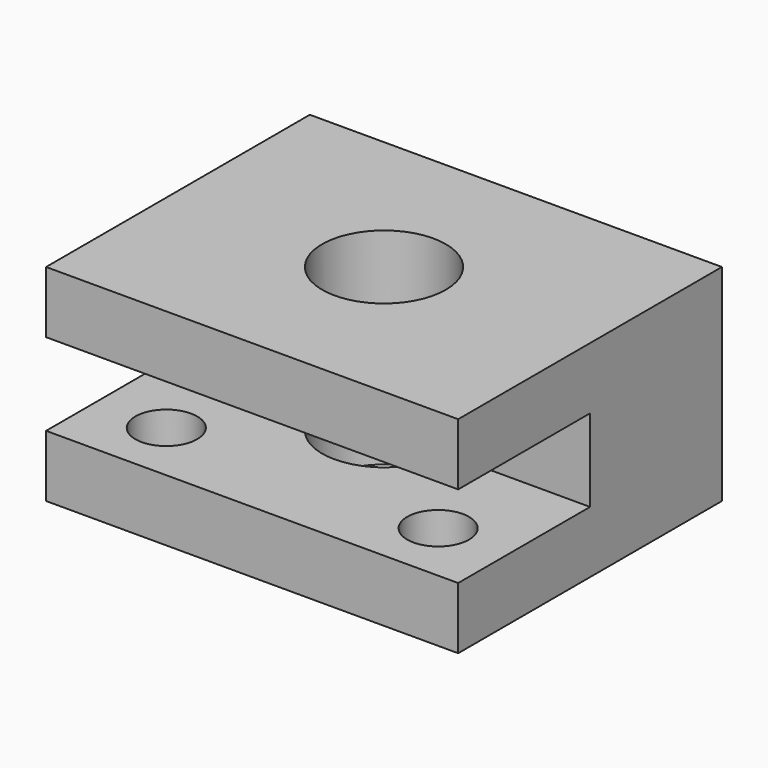
from build123d import *

# Parameters (mm, degrees)
F0_W     = 100
F0_H     = 80
F0_R     = 15
F1_DEPTH = 50
F2_W     = 120
F2_H     = 20
F3_DEPTH = 40
F4_R     = 7.5
F5_DEPTH = 25


with BuildPart() as f1:
    # F0 (on Top) → F1 (new body)
    with BuildSketch(Plane.XY):
        Rectangle(F0_W, F0_H)
        Circle(F0_R, mode=Mode.SUBTRACT)
    extrude(amount=F1_DEPTH)

    # F2 (on face) → F3 (cut)
    with BuildSketch(Plane.XZ.offset(40)):
        with Locations((3.9423131943, 25.000000596)):
            Rectangle(F2_W, F2_H)
    extrude(amount=-F3_DEPTH, mode=Mode.SUBTRACT)

    # F4 (on face) → F5 (cut)
    with BuildSketch(Plane.XY.offset(15.000000596)):
        with Locations((-32.9807698727, -24.8076934367)):
            Circle(F4_R)
        with Locations((32.9807698727, -24.8076934367)):
            Circle(F4_R)
    extrude(amount=-F5_DEPTH, mode=Mode.SUBTRACT)


solid = f1.part
